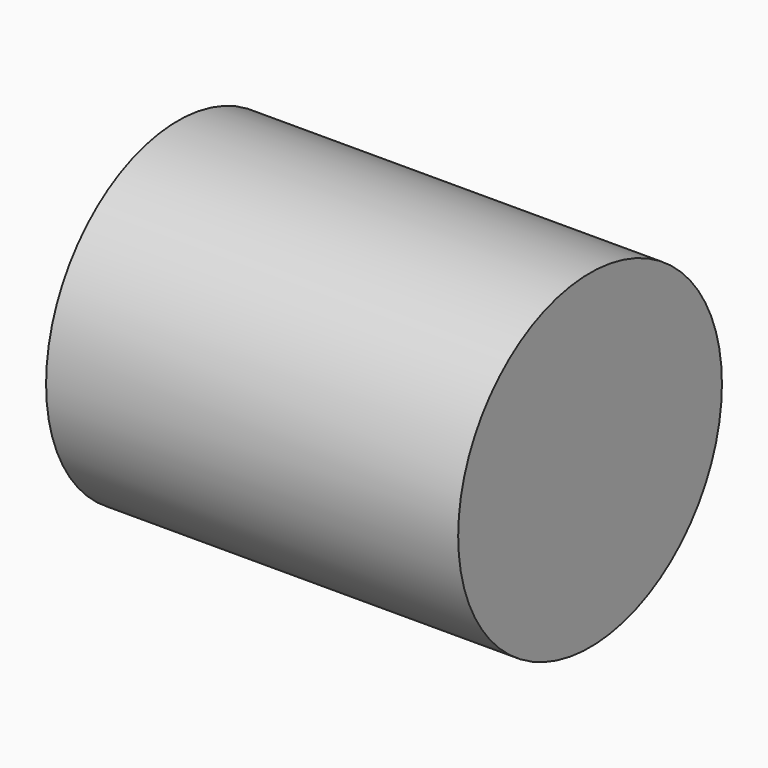
from build123d import *

# Parameters (mm, degrees)
F1_R     = 10
F2_DEPTH = 25


with BuildPart() as f2:
    # F1 (on face) → F2 (new body)
    with BuildSketch(Plane.YZ):
        Circle(F1_R)
    extrude(amount=F2_DEPTH)


solid = f2.part
